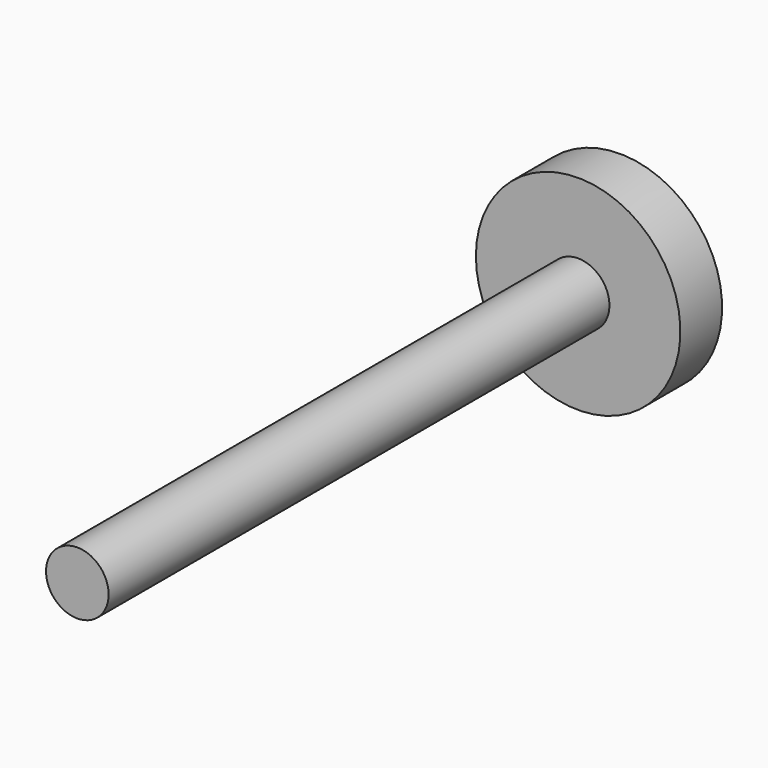
from build123d import *

# Parameters (mm, degrees)
F0_R     = 15
F1_DEPTH = 300
F2_R     = 49
F2_R_2   = 15
F3_DEPTH = 25


with BuildPart() as f1:
    # F0 (on Front) → F1 (new body)
    with BuildSketch(Plane.XZ):
        with Locations((-50.172239542, 22.9911319911)):
            Circle(F0_R)
    extrude(amount=F1_DEPTH)

    # F2 (on face) → F3 (join)
    with BuildSketch(Plane(origin=(0, 0, 0), x_dir=(-1, 0, 0), z_dir=(0, 1, 0))):
        with Locations((50.172239542, 22.9911319911)):
            Circle(F2_R)
        with Locations((50.172239542, 22.9911319911)):
            Circle(F2_R_2, mode=Mode.SUBTRACT)
        with Locations((50.172239542, 22.9911319911)):
            Circle(F2_R_2)
    extrude(amount=F3_DEPTH)


solid = f1.part
